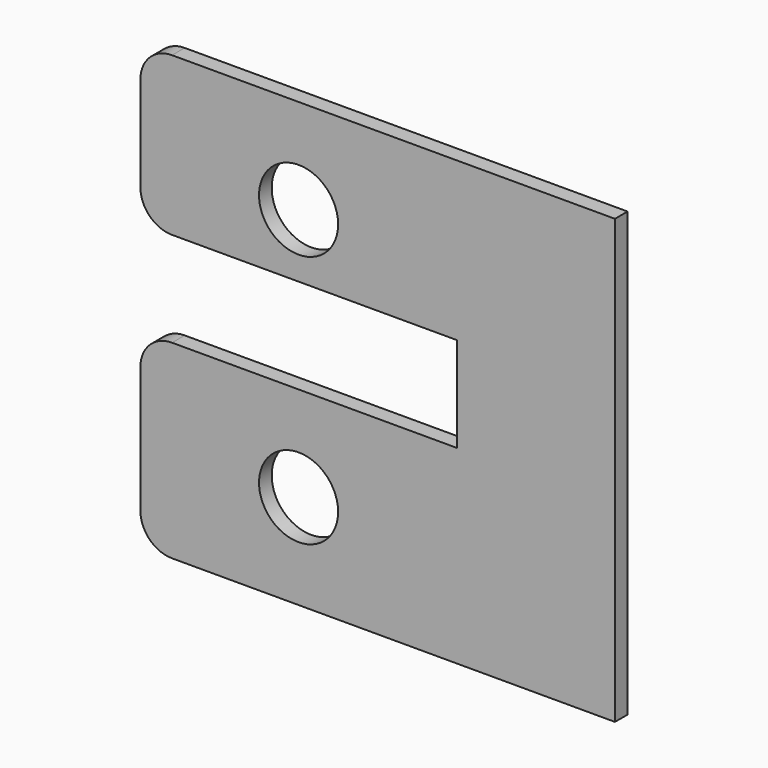
from build123d import *

# Parameters (mm, degrees)
F0_R     = 7.9375
F1_DEPTH = 3.175


# Not quite as in the source:
# - a feature names something its author has since deleted; it is built from what else it names


with BuildPart() as f1:
    # F0 (on Front) → F1 (new body)
    with BuildSketch(Plane.XZ):
        with BuildLine():
            Line((-107.95, 82.55), (-107.95, 63.5))
            ThreePointArc((-107.95, 63.5), (-106.0901280605, 59.0098719395), (-101.6, 57.15))
            Line((-101.6, 57.15), (-44.45, 57.15))
            Line((-44.45, 57.15), (-44.45, 88.9))
            Line((-44.45, 88.9), (-101.6, 88.9))
            ThreePointArc((-101.6, 88.9), (-106.0901280605, 87.0401280605), (-107.95, 82.55))
        make_face()
        with Locations((-76.2, 69.85)):
            Circle(F0_R, mode=Mode.SUBTRACT)
        Polygon((-44.45, 88.9), (-44.45, 57.15), (-44.45, 38.1), (-44.45, 0), (-12.7, 0), (-12.7, 88.9), align=None)
        with BuildLine():
            Line((-44.45, 0), (-44.45, 38.1))
            Line((-44.45, 38.1), (-101.6, 38.1))
            ThreePointArc((-101.6, 38.1), (-106.0901280605, 36.2401280605), (-107.95, 31.75))
            Line((-107.95, 31.75), (-107.95, 6.35))
            ThreePointArc((-107.95, 6.35), (-106.0901280605, 1.8598719395), (-101.6, 0))
            Line((-101.6, 0), (-95.25, 0))
            Line((-95.25, 0), (-44.45, 0))
        make_face()
        with Locations((-76.2, 19.05)):
            Circle(F0_R, mode=Mode.SUBTRACT)
    extrude(amount=F1_DEPTH)


solid = f1.part
